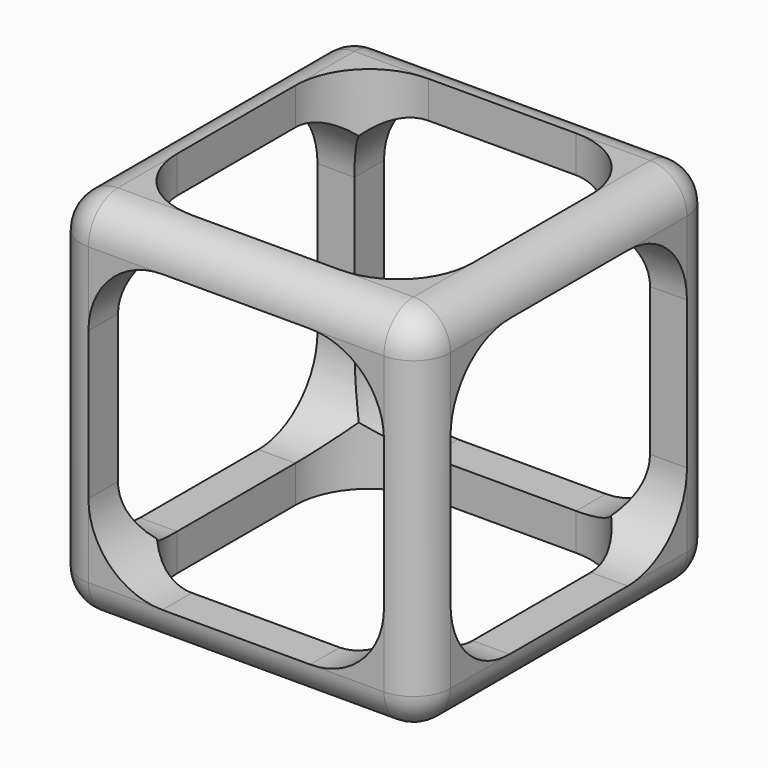
from build123d import *

# Parameters (mm, degrees)
F0_W     = 50
F0_H     = 50
F1_DEPTH = 50
F3_DEPTH = 50.001
F5_DEPTH = 50.001
F7_DEPTH = 50.001
F8_R     = 4.99999


# Not quite as in the source:
# - a fillet or chamfer is up to 0.001 mm smaller than in the source, because OpenCascade refuses the exact size


with BuildPart() as f1:
    # F0 (on Top) → F1 (new body)
    with BuildSketch(Plane.XY):
        Rectangle(F0_W, F0_H)
    extrude(amount=F1_DEPTH)

    # F2 (on face) → F3 (cut, through all)
    with BuildSketch(Plane.XY.offset(50)):
        with BuildLine():
            ThreePointArc((20, 10), (17.0710678119, 17.0710678119), (10, 20))
            Line((10, 20), (-10, 20))
            ThreePointArc((-10, 20), (-17.0710678119, 17.0710678119), (-20, 10))
            Line((-20, 10), (-20, -10))
            ThreePointArc((-20, -10), (-17.0710678119, -17.0710678119), (-10, -20))
            Line((-10, -20), (10, -20))
            ThreePointArc((10, -20), (17.0710678119, -17.0710678119), (20, -10))
            Line((20, -10), (20, 10))
        make_face()
    extrude(amount=-F3_DEPTH, mode=Mode.SUBTRACT)

    # F4 (on face) → F5 (cut, through all)
    with BuildSketch(Plane(origin=(-25, 0, 0), x_dir=(0, -1, 0), z_dir=(-1, 0, 0))):
        with BuildLine():
            Line((10, 45), (-10, 45))
            ThreePointArc((-10, 45), (-17.0710678119, 42.0710678119), (-20, 35))
            Line((-20, 35), (-20, 15))
            ThreePointArc((-20, 15), (-17.0710678119, 7.9289321881), (-10, 5))
            Line((-10, 5), (10, 5))
            ThreePointArc((10, 5), (17.0710678119, 7.9289321881), (20, 15))
            Line((20, 15), (20, 35))
            ThreePointArc((20, 35), (17.0710678119, 42.0710678119), (10, 45))
        make_face()
    extrude(amount=-F5_DEPTH, mode=Mode.SUBTRACT)

    # F6 (on face) → F7 (cut, through all)
    with BuildSketch(Plane.XZ.offset(25)):
        with BuildLine():
            Line((10, 45), (-10, 45))
            ThreePointArc((-10, 45), (-17.0710678119, 42.0710678119), (-20, 35))
            Line((-20, 35), (-20, 15))
            ThreePointArc((-20, 15), (-17.0710678119, 7.9289321881), (-10, 5))
            Line((-10, 5), (10, 5))
            ThreePointArc((10, 5), (17.0710678119, 7.9289321881), (20, 15))
            Line((20, 15), (20, 35))
            ThreePointArc((20, 35), (17.0710678119, 42.0710678119), (10, 45))
        make_face()
    extrude(amount=-F7_DEPTH, mode=Mode.SUBTRACT)

    # F8 (radius 5 in the source; OpenCascade refuses exactly that, so slightly less here)
    f8_edges = [f1.edges().sort_by_distance(p)[0] for p in [
        (0, 25, 0),
        (-25, 0, 0),
        (0, -25, 0),
        (25, 0, 0),
        (25, 25, 25),
        (-25, 25, 25),
        (-25, -25, 25),
        (0, 25, 50),
        (-25, 0, 50),
        (0, -25, 50),
        (25, 0, 50),
        (25, -25, 25),
    ]]
    fillet(f8_edges, radius=F8_R)


solid = f1.part
